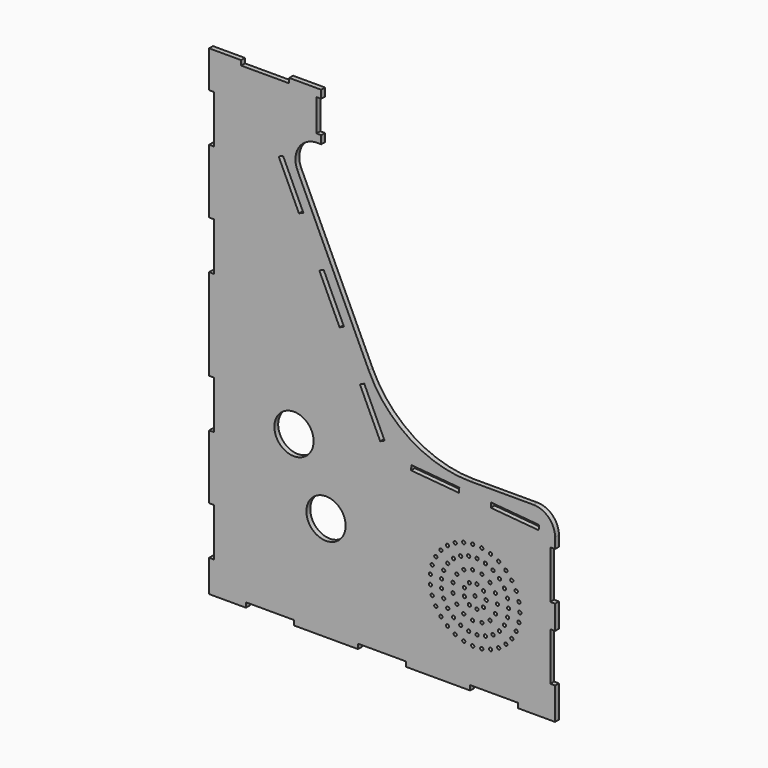
from build123d import *

# Parameters (mm, degrees)
F1_DEPTH = 3
F2_R     = 12.25
F3_DEPTH = 3
F4_R     = 13.5
F5_R     = 70
F6_R     = 1
F7_DEPTH = 3


# Not quite as in the source:
# - a feature names something its author has since deleted; it is built from what else it names


with BuildPart() as f1:
    # F0 (on Front) → F1 (new body)
    with BuildSketch(Plane.XZ):
        Polygon((0, 20), (0, 0), (23, 0), (23, 3), (53, 3), (53, 0), (93, 0), (93, 3), (123, 3), (123, 0), (163, 0), (163, 3), (193, 3), (193, 0), (216, 0), (216, 20), (213, 20), (213, 50), (216, 50), (216, 65), (213, 65), (213, 95), (216, 95), (216, 115), (118.5, 115), (46.222312986, 270), (70, 270), (70, 275), (67, 275), (67, 295), (70, 295), (70, 300), (50, 300), (50, 297), (20, 297), (20, 300), (0, 300), (0, 277), (3, 277), (3, 247), (0, 247), (0, 207), (3, 207), (3, 177), (0, 177), (0, 120), (3, 120), (3, 90), (0, 90), (0, 50), (3, 50), (3, 20), align=None)
    extrude(amount=F1_DEPTH)

    # F2 (on face) → F3 (cut, through all)
    with BuildSketch(Plane.XZ.offset(3)):
        Polygon((156.2169022088, 109.3853277176), (126.331061266, 112), (126.0695940378, 109.0114159057), (155.9554349805, 106.3967436233), align=None)
        Polygon((206.0266371134, 105.0275405802), (176.1407961706, 107.6422128626), (175.8793289424, 104.6536287683), (205.7651698851, 102.0389564859), align=None)
        Polygon((84.1967806423, 174.3662818095), (71.51823279, 201.5555154206), (68.7993094289, 200.2876606354), (81.4778572811, 173.0984270243), align=None)
        Polygon((109.5538763467, 119.9878145873), (96.8753284945, 147.1770481984), (94.1564051334, 145.9091934132), (106.8349529856, 118.7199598021), align=None)
        Polygon((56.1207615767, 227.4768942465), (58.8396849378, 228.7447490317), (46.1611370856, 255.9339826428), (43.4422137245, 254.6661278576), align=None)
        with Locations((73, 65.25)):
            Circle(F2_R)
        with Locations((53, 105.25)):
            Circle(F2_R)
    extrude(amount=-F3_DEPTH, mode=Mode.SUBTRACT)

    # F4
    f4_edges = [f1.edges().sort_by_distance(p)[0] for p in [
        (216, -1.5, 115),
        (46.222313, -1.5, 270),
    ]]
    fillet(f4_edges, radius=F4_R)

    # F5
    f5_edges = [f1.edges().sort_by_distance(p)[0] for p in [
        (118.5, -1.5, 115),
    ]]
    fillet(f5_edges, radius=F5_R)

    # F6 (on face) → F7 (cut, through all)
    with BuildSketch(Plane.XZ.offset(3)):
        with Locations((166, 53)):
            Circle(F6_R)
        with Locations((173, 53)):
            Circle(F6_R)
        with Locations((180, 53)):
            Circle(F6_R)
        with Locations((187, 53)):
            Circle(F6_R)
        with Locations((171.3623111018, 57.4995132678)):
            Circle(F6_R)
        with Locations((167.2155372437, 59.8936542711)):
            Circle(F6_R)
        with Locations((162.5, 59.0621778265)):
            Circle(F6_R)
        with Locations((159.4221516545, 55.3941410033)):
            Circle(F6_R)
        with Locations((159.4221516545, 50.6058589967)):
            Circle(F6_R)
        with Locations((162.5, 46.9378221735)):
            Circle(F6_R)
        with Locations((167.2155372437, 46.1063457289)):
            Circle(F6_R)
        with Locations((178.789636407, 58.6943130031)):
            Circle(F6_R)
        with Locations((175.367828489, 63.4040275567)):
            Circle(F6_R)
        with Locations((170.3262379212, 66.3147912281)):
            Circle(F6_R)
        with Locations((164.5366015143, 66.9233065352)):
            Circle(F6_R)
        with Locations((159, 65.124355653)):
            Circle(F6_R)
        with Locations((154.6737620788, 61.2289935321)):
            Circle(F6_R)
        with Locations((152.3059335897, 55.9107636714)):
            Circle(F6_R)
        with Locations((152.3059335897, 50.0892363286)):
            Circle(F6_R)
        with Locations((154.6737620788, 44.7710064679)):
            Circle(F6_R)
        with Locations((159, 40.875644347)):
            Circle(F6_R)
        with Locations((164.5366015143, 39.0766934648)):
            Circle(F6_R)
        with Locations((170.3262379212, 39.6852087719)):
            Circle(F6_R)
        with Locations((175.367828489, 42.5959724433)):
            Circle(F6_R)
        with Locations((178.789636407, 47.3056869969)):
            Circle(F6_R)
        with Locations((186.3402463837, 58.2224876305)):
            Circle(F6_R)
        with Locations((184.4024402809, 63.1168271561)):
            Circle(F6_R)
        with Locations((181.3083411758, 67.3754892245)):
            Circle(F6_R)
        with Locations((177.2523626946, 70.7308864355)):
            Circle(F6_R)
        with Locations((172.4893568819, 72.9721868422)):
            Circle(F6_R)
        with Locations((167.3186009101, 73.958561297)):
            Circle(F6_R)
        with Locations((162.0649923937, 73.6280322653)):
            Circle(F6_R)
        with Locations((157.0586348771, 72.0013681018)):
            Circle(F6_R)
        with Locations((152.6140962153, 69.1807780983)):
            Circle(F6_R)
        with Locations((149.0106431181, 65.3434902981)):
            Circle(F6_R)
        with Locations((146.4746937963, 60.7306156064)):
            Circle(F6_R)
        with Locations((145.1655912724, 55.6319979049)):
            Circle(F6_R)
        with Locations((145.1655912724, 50.3680020951)):
            Circle(F6_R)
        with Locations((146.4746937963, 45.2693843936)):
            Circle(F6_R)
        with Locations((149.0106431181, 40.6565097019)):
            Circle(F6_R)
        with Locations((152.6140962153, 36.8192219017)):
            Circle(F6_R)
        with Locations((157.0586348771, 33.9986318982)):
            Circle(F6_R)
        with Locations((162.0649923937, 32.3719677347)):
            Circle(F6_R)
        with Locations((167.3186009101, 32.041438703)):
            Circle(F6_R)
        with Locations((172.4893568819, 33.0278131578)):
            Circle(F6_R)
        with Locations((177.2523626946, 35.2691135645)):
            Circle(F6_R)
        with Locations((181.3083411758, 38.6245107755)):
            Circle(F6_R)
        with Locations((184.4024402809, 42.8831728439)):
            Circle(F6_R)
        with Locations((186.3402463837, 47.7775123695)):
            Circle(F6_R)
        with Locations((194, 53)):
            Circle(F6_R)
        with Locations((193.4268383551, 58.6363585625)):
            Circle(F6_R)
        with Locations((191.7308187254, 64.0419639432)):
            Circle(F6_R)
        with Locations((188.9813763538, 68.9955100227)):
            Circle(F6_R)
        with Locations((185.2910737341, 73.2941980424)):
            Circle(F6_R)
        with Locations((180.8109922892, 76.7620392099)):
            Circle(F6_R)
        with Locations((175.7245470797, 79.2570597001)):
            Circle(F6_R)
        with Locations((170.2399777701, 80.6771130812)):
            Circle(F6_R)
        with Locations((164.5818232725, 80.9640622008)):
            Circle(F6_R)
        with Locations((158.9817290968, 80.1061593283)):
            Circle(F6_R)
        with Locations((153.6689637564, 78.138527108)):
            Circle(F6_R)
        with Locations((148.8610324887, 75.1417206343)):
            Circle(F6_R)
        with Locations((144.7547725646, 71.2384295162)):
            Circle(F6_R)
        with Locations((141.518294748, 66.5884549509)):
            Circle(F6_R)
        with Locations((139.2841008208, 61.3821674433)):
            Circle(F6_R)
        with Locations((138.143658945, 55.8327130156)):
            Circle(F6_R)
        with Locations((138.143658945, 50.1672869844)):
            Circle(F6_R)
        with Locations((139.2841008208, 44.6178325567)):
            Circle(F6_R)
        with Locations((141.518294748, 39.4115450491)):
            Circle(F6_R)
        with Locations((144.7547725646, 34.7615704838)):
            Circle(F6_R)
        with Locations((148.8610324887, 30.8582793657)):
            Circle(F6_R)
        with Locations((153.6689637564, 27.861472892)):
            Circle(F6_R)
        with Locations((158.9817290968, 25.8938406717)):
            Circle(F6_R)
        with Locations((164.5818232725, 25.0359377992)):
            Circle(F6_R)
        with Locations((170.2399777701, 25.3228869188)):
            Circle(F6_R)
        with Locations((175.7245470797, 26.7429402999)):
            Circle(F6_R)
        with Locations((180.8109922892, 29.2379607901)):
            Circle(F6_R)
        with Locations((185.2910737341, 32.7058019576)):
            Circle(F6_R)
        with Locations((188.9813763538, 37.0044899773)):
            Circle(F6_R)
        with Locations((191.7308187254, 41.9580360568)):
            Circle(F6_R)
        with Locations((193.4268383551, 47.3636414375)):
            Circle(F6_R)
        with Locations((171.3623111018, 48.5004867322)):
            Circle(F6_R)
    extrude(amount=-F7_DEPTH, mode=Mode.SUBTRACT)


solid = f1.part
